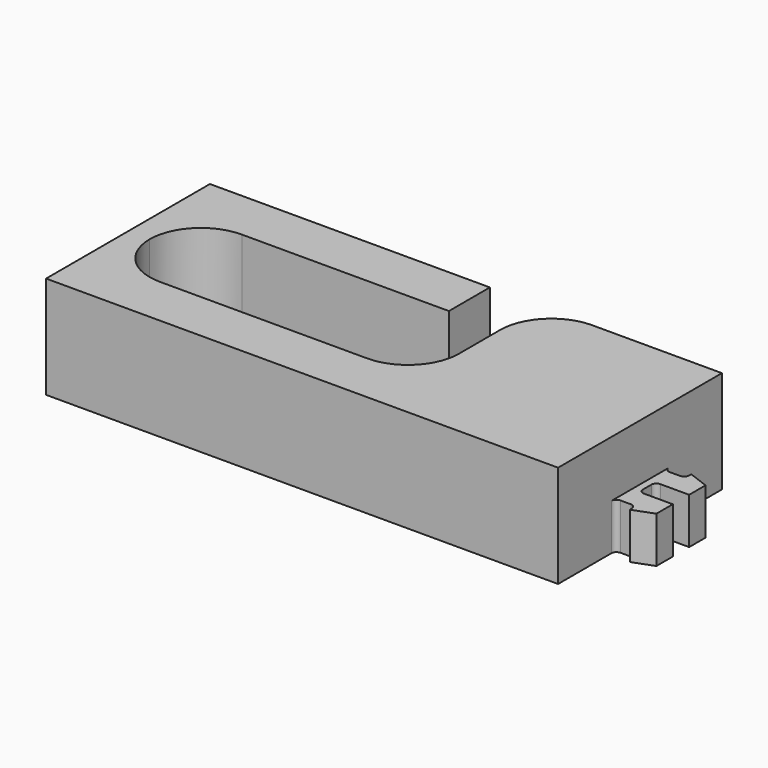
from build123d import *

# Parameters (mm, degrees)
F0_W     = 10.7198789741
F0_H     = 5
F1_DEPTH = 10
F0_W_2   = 2
F0_H_2   = 2
F0_W_3   = 0.7
F2_DEPTH = 4.5
F3_R     = 4.99999
F4_R     = 0.5


# Not quite as in the source:
# - a fillet or chamfer is up to 0.001 mm smaller than in the source, because OpenCascade refuses the exact size


with BuildPart() as f1:
    # F0 (on Top) → F1 (new body)
    with BuildSketch(Plane.XY):
        Polygon((-10.9434188306, 20), (-10.9434188306, 0), (5.6756753474, 0), (5.6756753474, 5), (-8.8288290426, 5), (-8.8288290426, 15), (5.6756753474, 15), (5.6756753474, 20), align=None)
        Polygon((5.6756753474, 5), (5.6756753474, 0), (39.0565811694, 0), (39.0565811694, 7), (39.0565811694, 9), (39.0565811694, 11), (39.0565811694, 13), (39.0565811694, 20), (21.3955543215, 20), (21.3955543215, 15), (21.3955543215, 5), align=None)
        with Locations((11.0356148345, 17.5)):
            Rectangle(F0_W, F0_H)
    extrude(amount=F1_DEPTH)

    # F0 (on Top) → F2 (join)
    with BuildSketch(Plane.XY):
        Polygon((39.0565811694, 9), (39.0565811694, 7), (41.0565811694, 7), (41.0565811694, 9), (39.7565811694, 9), align=None)
        with Locations((42.0565811694, 8)):
            Rectangle(F0_W_2, F0_H_2)
        Polygon((43.0565811694, 7), (41.0565811694, 7), (41.0565811694, 6.25), align=None)
        Polygon((39.0565811694, 13), (39.0565811694, 11), (39.7565811694, 11), (41.0565811694, 11), (41.0565811694, 13), align=None)
        with Locations((42.0565811694, 12)):
            Rectangle(F0_W_2, F0_H_2)
        Polygon((41.0565811694, 13.75), (41.0565811694, 13), (43.0565811694, 13), align=None)
        with Locations((39.4065811694, 10)):
            Rectangle(F0_W_3, F0_H_2)
    extrude(amount=F2_DEPTH)

    # F3 (radius 5 in the source; OpenCascade refuses exactly that, so slightly less here)
    f3_edges = [f1.edges().sort_by_distance(p)[0] for p in [
        (-8.828829, 15, 5),
        (-8.828829, 5, 5),
        (21.395554, 5, 5),
        (21.395554, 20, 5),
    ]]
    fillet(f3_edges, radius=F3_R)

    # F4
    f4_edges = [f1.edges().sort_by_distance(p)[0] for p in [
        (39.056581, 13, 2.25),
        (39.056581, 7, 2.25),
        (41.056581, 7, 2.25),
        (41.056581, 13, 2.25),
        (39.756581, 11, 2.25),
        (39.756581, 9, 2.25),
    ]]
    fillet(f4_edges, radius=F4_R)


solid = f1.part
